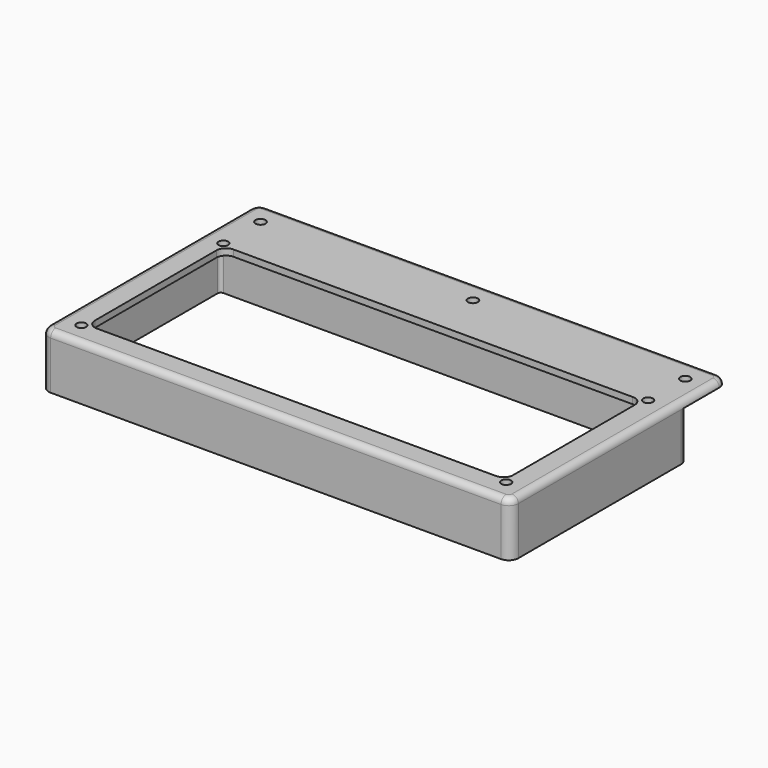
from build123d import *

# Parameters (mm, degrees)
F2_DEPTH = 17
F3_T     = -2
F1_R     = 1.55
F4_DEPTH = 2
F5_DEPTH = 25
F6_D     = 3
F7_R     = 1.99999


# Not quite as in the source:
# - a fillet or chamfer is up to 0.001 mm smaller than in the source, because OpenCascade refuses the exact size


with BuildPart() as f2:
    # F1 (on Top) → F2 (new body)
    with BuildSketch(Plane.XY):
        with BuildLine():
            ThreePointArc((73.2924652381, 31.6927541938), (72.4137855817, 33.8140745374), (70.2924652381, 34.6927541938))
            Line((70.2924652381, 34.6927541938), (-70.2924652381, 34.6927541938))
            ThreePointArc((-70.2924652381, 34.6927541938), (-72.4137855817, 33.8140745374), (-73.2924652381, 31.6927541938))
            Line((-73.2924652381, 31.6927541938), (-73.2924652381, -31.6927541938))
            ThreePointArc((-73.2924652381, -31.6927541938), (-72.4137855817, -33.8140745374), (-70.2924652381, -34.6927541938))
            Line((-70.2924652381, -34.6927541938), (70.2924652381, -34.6927541938))
            ThreePointArc((70.2924652381, -34.6927541938), (72.4137855817, -33.8140745374), (73.2924652381, -31.6927541938))
            Line((73.2924652381, -31.6927541938), (73.2924652381, 31.6927541938))
        make_face()
        with BuildLine():
            ThreePointArc((65.2924652381, -23.6927541938), (64.4137855817, -25.8140745374), (62.2924652381, -26.6927541938))
            Line((62.2924652381, -26.6927541938), (-62.2924652381, -26.6927541938))
            ThreePointArc((-62.2924652381, -26.6927541938), (-64.4137855817, -25.8140745374), (-65.2924652381, -23.6927541938))
            Line((-65.2924652381, -23.6927541938), (-65.2924652381, 23.6927541938))
            ThreePointArc((-65.2924652381, 23.6927541938), (-64.4137855817, 25.8140745374), (-62.2924652381, 26.6927541938))
            Line((-62.2924652381, 26.6927541938), (62.2924652381, 26.6927541938))
            ThreePointArc((62.2924652381, 26.6927541938), (64.4137855817, 25.8140745374), (65.2924652381, 23.6927541938))
            Line((65.2924652381, 23.6927541938), (65.2924652381, -23.6927541938))
        make_face(mode=Mode.SUBTRACT)
        with BuildLine():
            Line((-62.2924652381, -26.6927541938), (62.2924652381, -26.6927541938))
            ThreePointArc((62.2924652381, -26.6927541938), (64.4137855817, -25.8140745374), (65.2924652381, -23.6927541938))
            Line((65.2924652381, -23.6927541938), (65.2924652381, 23.6927541938))
            ThreePointArc((65.2924652381, 23.6927541938), (64.4137855817, 25.8140745374), (62.2924652381, 26.6927541938))
            Line((62.2924652381, 26.6927541938), (-62.2924652381, 26.6927541938))
            ThreePointArc((-62.2924652381, 26.6927541938), (-64.4137855817, 25.8140745374), (-65.2924652381, 23.6927541938))
            Line((-65.2924652381, 23.6927541938), (-65.2924652381, -23.6927541938))
            ThreePointArc((-65.2924652381, -23.6927541938), (-64.4137855817, -25.8140745374), (-62.2924652381, -26.6927541938))
        make_face()
    extrude(amount=-F2_DEPTH)

    # F3
    f3_openings = [f2.faces().sort_by_distance(p)[0] for p in [
        (0, 0, -17),
    ]]
    offset(amount=F3_T, openings=f3_openings)

    # F1 (on Top) → F4 (join)
    with BuildSketch(Plane.XY):
        with BuildLine():
            Line((-70.2924652381, 34.6927541938), (70.2924652381, 34.6927541938))
            ThreePointArc((70.2924652381, 34.6927541938), (72.4137855817, 33.8140745374), (73.2924652381, 31.6927541938))
            Line((73.2924652381, 31.6927541938), (73.2924652381, 34.6927541938))
            Line((73.2924652381, 34.6927541938), (73.2924652381, 46.6927541938))
            ThreePointArc((73.2924652381, 46.6927541938), (72.4137855817, 48.8140745374), (70.2924652381, 49.6927541938))
            Line((70.2924652381, 49.6927541938), (-70.2924652381, 49.6927541938))
            ThreePointArc((-70.2924652381, 49.6927541938), (-72.4137855817, 48.8140745374), (-73.2924652381, 46.6927541938))
            Line((-73.2924652381, 46.6927541938), (-73.2924652381, 34.6927541938))
            Line((-73.2924652381, 34.6927541938), (-73.2924652381, 31.6927541938))
            ThreePointArc((-73.2924652381, 31.6927541938), (-72.4137855817, 33.8140745374), (-70.2924652381, 34.6927541938))
        make_face()
        with Locations((-66.2924652381, 42.1927541938)):
            Circle(F1_R, mode=Mode.SUBTRACT)
        with Locations((0, 42.1927541938)):
            Circle(F1_R, mode=Mode.SUBTRACT)
        with Locations((66.2924652381, 42.1927541938)):
            Circle(F1_R, mode=Mode.SUBTRACT)
    extrude(amount=-F4_DEPTH)

    # F1 (on Top) → F5 (cut)
    with BuildSketch(Plane.XY):
        with BuildLine():
            Line((-62.2924652381, -26.6927541938), (62.2924652381, -26.6927541938))
            ThreePointArc((62.2924652381, -26.6927541938), (64.4137855817, -25.8140745374), (65.2924652381, -23.6927541938))
            Line((65.2924652381, -23.6927541938), (65.2924652381, 23.6927541938))
            ThreePointArc((65.2924652381, 23.6927541938), (64.4137855817, 25.8140745374), (62.2924652381, 26.6927541938))
            Line((62.2924652381, 26.6927541938), (-62.2924652381, 26.6927541938))
            ThreePointArc((-62.2924652381, 26.6927541938), (-64.4137855817, 25.8140745374), (-65.2924652381, 23.6927541938))
            Line((-65.2924652381, 23.6927541938), (-65.2924652381, -23.6927541938))
            ThreePointArc((-65.2924652381, -23.6927541938), (-64.4137855817, -25.8140745374), (-62.2924652381, -26.6927541938))
        make_face()
    extrude(amount=-F5_DEPTH, mode=Mode.SUBTRACT)

    # F6 (through all)
    with Locations(Plane.XY):
        with Locations((-66.2924652381, 27.6927541938), (66.2980739571, 27.6781461437), (66.291973394, -27.6938535203), (-66.2985658012, -27.6792454701)):
            Hole(F6_D / 2)

    # F7 (radius 2 in the source; OpenCascade refuses exactly that, so slightly less here)
    f7_edges = [f2.edges().sort_by_distance(p)[0] for p in [
        (-73.292465, 7.5, 0),
    ]]
    fillet(f7_edges, radius=F7_R)


solid = f2.part
